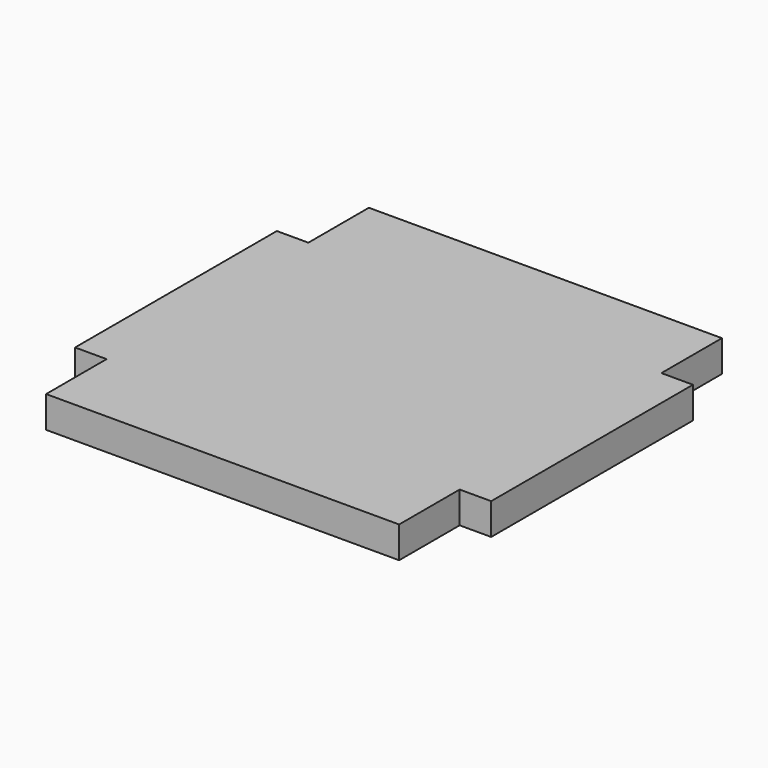
from build123d import *

# Parameters (mm, degrees)
F0_W     = 35.56
F0_H     = 40.64
F1_DEPTH = 3.175
F2_W     = 25.4
F2_H     = 3.175
F3_DEPTH = 3.175
F4_W     = 25.4
F4_H     = 3.175
F5_DEPTH = 3.175


# Not quite as in the source:
# - a length typed as a fraction of an inch, garbled in the dataset ("3 / 203.2 mm" for 3/8 in), is restored


with BuildPart() as f1:
    # F0 (on Top) → F1 (new body)
    with BuildSketch(Plane.XY):
        Rectangle(F0_W, F0_H)
    extrude(amount=F1_DEPTH)

    # F2 (on face) → F3 (join)
    with BuildSketch(Plane(origin=(-17.78, 0, 0), x_dir=(0, -1, 0), z_dir=(-1, 0, 0))):
        with Locations((0, 1.5875)):
            Rectangle(F2_W, F2_H)
    extrude(amount=F3_DEPTH)

    # F4 (on face) → F5 (join)
    with BuildSketch(Plane.YZ.offset(17.78)):
        with Locations((0, 1.5875)):
            Rectangle(F4_W, F4_H)
    extrude(amount=F5_DEPTH)


solid = f1.part
